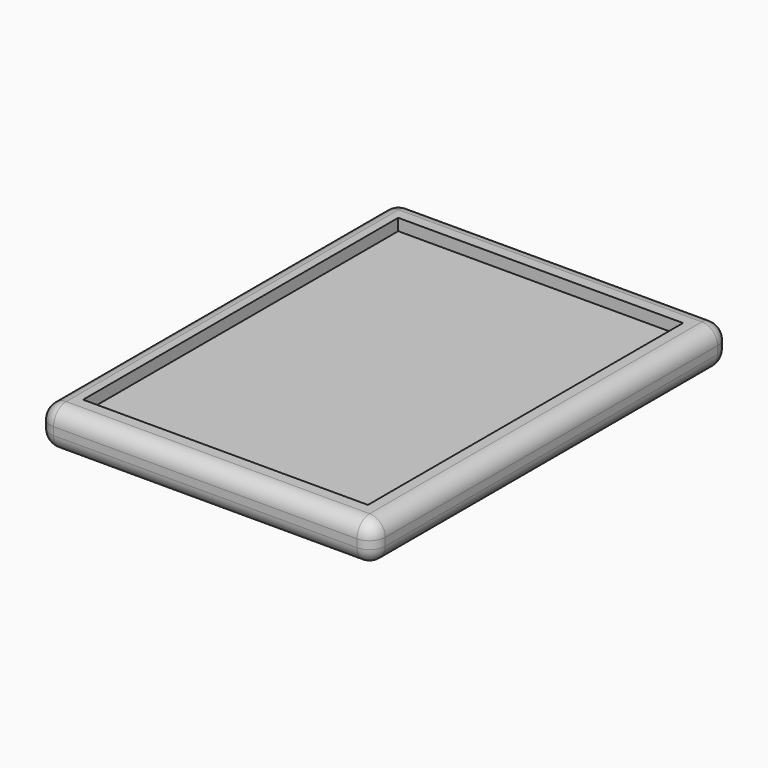
from build123d import *

# Parameters (mm, degrees)
F0_W         = 108.4600649774
F0_H         = 144.723303616
F1_DEPTH     = 12.7
F2_W         = 92.2743044794
F2_H         = 127.6071891189
F3_DEPTH     = 3.81
F4_R         = 5.08
F5_T1_DEPTH  = 20.32
F5_S5_W      = 5.08
F5_S5_H      = 5.08
F5_T6_DEPTH  = 5.08
F5_S11_W     = 5.08
F5_S11_H     = 5.08
F5_T12_DEPTH = 5.08
F5_S17_W     = 5.08
F5_S17_H     = 5.08
F5_T18_DEPTH = 5.08
F5_S23_W     = 5.08
F5_S23_H     = 5.08
F5_T24_DEPTH = 5.08
F7_DEPTH     = 5.08
F8_DEPTH     = 5.08
F9_R         = 5.08


# Not quite as in the source:
# - a fillet or chamfer that OpenCascade refuses, or shapes differently, is made with other operations: its cross-section is extruded or revolved along the edge and cut away or added


with BuildPart() as f1:
    # F0 (on Top) → F1 (new body)
    with BuildSketch(Plane.XY):
        with Locations((1.0477285832, -0.3120861948)):
            Rectangle(F0_W, F0_H)
    extrude(amount=F1_DEPTH)

    # F2 (on face) → F3 (cut, symmetric)
    with BuildSketch(Plane.XY.offset(12.7)):
        with Locations((0.7300172001, -0.29200688)):
            Rectangle(F2_W, F2_H)
    extrude(amount=F3_DEPTH, both=True, mode=Mode.SUBTRACT)

    # F4
    f4_edges = [f1.edges().sort_by_distance(p)[0] for p in [
        (1.047729, 72.049566, 12.7),
        (-53.182304, -0.312086, 12.7),
        (55.277761, -0.312086, 12.7),
        (1.047729, -72.673738, 12.7),
    ]]
    fillet(f4_edges, radius=F4_R)

    # F5: fillet of radius 5.08 on 4 edges, made by hand

    # F5_s2 → F5_t1 (cut)
    with BuildSketch(Plane.XY.offset(-12.7)):
        with BuildLine():
            ThreePointArc((-48.1023039055, 72.0495656133), (-51.6944063539, 70.5616680617), (-53.1823039055, 66.9695656133))
            Line((-53.1823039055, 66.9695656133), (-53.1823039055, 72.0495656133))
            Line((-53.1823039055, 72.0495656133), (-48.1023039055, 72.0495656133))
        make_face()
        with BuildLine():
            ThreePointArc((55.2777610719, -67.5937380028), (53.7898635203, -71.1858404512), (50.1977610719, -72.6737380028))
            Line((50.1977610719, -72.6737380028), (55.2777610719, -72.6737380028))
            Line((55.2777610719, -72.6737380028), (55.2777610719, -67.5937380028))
        make_face()
        with BuildLine():
            ThreePointArc((50.1977610719, 72.0495656133), (53.7898635203, 70.5616680617), (55.2777610719, 66.9695656133))
            Line((55.2777610719, 66.9695656133), (55.2777610719, 72.0495656133))
            Line((55.2777610719, 72.0495656133), (50.1977610719, 72.0495656133))
        make_face()
        with BuildLine():
            ThreePointArc((-53.1823039055, -67.5937380028), (-51.6944063539, -71.1858404512), (-48.1023039055, -72.6737380028))
            Line((-48.1023039055, -72.6737380028), (-53.1823039055, -72.6737380028))
            Line((-53.1823039055, -72.6737380028), (-53.1823039055, -67.5937380028))
        make_face()
    extrude(amount=F5_T1_DEPTH, mode=Mode.SUBTRACT)


with BuildPart() as f5_tool4:
    # F5_s5 → F5_t6 (new body)
    with BuildSketch(Plane.YZ.offset(-48.1023039055)):
        with Locations((-70.1337380028, 10.16)):
            Rectangle(F5_S5_W, F5_S5_H)
    extrude(amount=-F5_T6_DEPTH)

    # F5_s7 → F5_t8 (revolve, cut)
    with BuildSketch(Plane(origin=(-48.1023039055, -67.5937380028, 7.62), x_dir=(0, 0.7071067812, -0.7071067812), z_dir=(0, 0.7071067812, 0.7071067812))):
        with BuildLine():
            ThreePointArc((0, -5.08), (5.08, 0), (0, 5.08))
            Line((0, 5.08), (0, -5.08))
        make_face()
    revolve(axis=Axis((-48.1023039055, -67.5937380028, 7.62), (-1, 0, 0)), mode=Mode.SUBTRACT)


with BuildPart() as f1_1:
    add(f1.part)

    # F5_t3: cut F5_tool4
    add(f5_tool4.part, mode=Mode.SUBTRACT)


with BuildPart() as f5_tool10:
    # F5_s11 → F5_t12 (new body)
    with BuildSketch(Plane.XZ.offset(-66.9695656133)):
        with Locations((52.7377610719, 10.16)):
            Rectangle(F5_S11_W, F5_S11_H)
    extrude(amount=-F5_T12_DEPTH)

    # F5_s13 → F5_t14 (revolve, cut)
    with BuildSketch(Plane(origin=(50.1977610719, 66.9695656133, 7.62), x_dir=(-0.7071067812, 0, -0.7071067812), z_dir=(0.7071067812, 0, -0.7071067812))):
        with BuildLine():
            ThreePointArc((0, -5.08), (5.08, 0), (0, 5.08))
            Line((0, 5.08), (0, -5.08))
        make_face()
    revolve(axis=Axis((50.1977610719, 66.9695656133, 7.62), (0, 1, 0)), mode=Mode.SUBTRACT)


with BuildPart() as f1_2:
    add(f1_1.part)

    # F5_t9: cut F5_tool10
    add(f5_tool10.part, mode=Mode.SUBTRACT)


with BuildPart() as f5_tool16:
    # F5_s17 → F5_t18 (new body)
    with BuildSketch(Plane.YZ.offset(50.1977610719)):
        with Locations((-70.1337380028, 10.16)):
            Rectangle(F5_S17_W, F5_S17_H)
    extrude(amount=F5_T18_DEPTH)

    # F5_s19 → F5_t20 (revolve, cut)
    with BuildSketch(Plane(origin=(50.1977610719, -67.5937380028, 7.62), x_dir=(0, 0.7071067812, -0.7071067812), z_dir=(0, -0.7071067812, -0.7071067812))):
        with BuildLine():
            ThreePointArc((0, -5.08), (5.08, 0), (0, 5.08))
            Line((0, 5.08), (0, -5.08))
        make_face()
    revolve(axis=Axis((50.1977610719, -67.5937380028, 7.62), (1, 0, 0)), mode=Mode.SUBTRACT)


with BuildPart() as f1_3:
    add(f1_2.part)

    # F5_t15: cut F5_tool16
    add(f5_tool16.part, mode=Mode.SUBTRACT)


with BuildPart() as f5_tool22:
    # F5_s23 → F5_t24 (new body)
    with BuildSketch(Plane.XZ.offset(-66.9695656133)):
        with Locations((-50.6423039055, 10.16)):
            Rectangle(F5_S23_W, F5_S23_H)
    extrude(amount=-F5_T24_DEPTH)

    # F5_s25 → F5_t26 (revolve, cut)
    with BuildSketch(Plane(origin=(-48.1023039055, 66.9695656133, 7.62), x_dir=(0.7071067812, 0, -0.7071067812), z_dir=(0.7071067812, 0, 0.7071067812))):
        with BuildLine():
            ThreePointArc((0, -5.08), (5.08, 0), (0, 5.08))
            Line((0, 5.08), (0, -5.08))
        make_face()
    revolve(axis=Axis((-48.1023039055, 66.9695656133, 7.62), (0, 1, 0)), mode=Mode.SUBTRACT)


with BuildPart() as f1_4:
    add(f1_3.part)

    # F5_t21: cut F5_tool22
    add(f5_tool22.part, mode=Mode.SUBTRACT)

    # F6 (on face) → F7 (cut)
    with BuildSketch(Plane(origin=(0, 0, 0), x_dir=(1, 0, 0), z_dir=(0, 0, -1))):
        Polygon((3.4059861085, 7.1879082529), (-20.5314729904, -16.2908951516), (-9.6110993139, 46.108120036), (-34.5313920437, 46.108120036), (-35.3613404431, 41.5870853339), (-29.0712052055, 39.9490292824), (-45.1023137626, -50.8866389588), (-26.7560859861, -50.8866389588), (-22.1040067999, -24.7432643772), (-14.7436749419, -19.9601407069), (-3.4083270657, -50.8866389588), (18.0174460877, -50.8866389588), (18.781872245, -46.3874450041), (13.3216854068, -44.7493889526), (-1.8357932562, -8.0132519048), (14.7413339847, 7.2752712423), (21.0314692224, 8.7604420623), (21.7740546324, 13.2814767644), (-1.7047487721, 13.2814767644), (-2.4473341821, 8.7604420623), align=None)
    extrude(amount=-F7_DEPTH, mode=Mode.SUBTRACT)

    # F6 (on face) → F8 (cut)
    with BuildSketch(Plane(origin=(0, 0, 0), x_dir=(1, 0, 0), z_dir=(0, 0, -1))):
        with BuildLine():
            add(Edge.make_bspline(
                [(35.2279550018, -52.874146968), (30.5103535736, -52.874146968), (27.2014803496, -49.598034865)],
                knots=[0, 0, 0, 1, 1, 1], degree=2))
            add(Edge.make_bspline(
                [(43.2653500278, -49.5543533703), (39.9892379248, -52.874146968), (35.2279550018, -52.874146968)],
                knots=[0, 0, 0, 1, 1, 1], degree=2))
            add(Edge.make_bspline(
                [(46.5414621307, -41.5387990917), (46.5414621307, -46.2345597726), (43.2653500278, -49.5543533703)],
                knots=[0, 0, 0, 1, 1, 1], degree=2))
            add(Edge.make_bspline(
                [(43.2325889067, -33.4795633185), (46.5414621307, -36.7556754214), (46.5414621307, -41.5387990917)],
                knots=[0, 0, 0, 1, 1, 1], degree=2))
            add(Edge.make_bspline(
                [(35.2279550018, -30.2034512155), (39.9237156827, -30.2034512155), (43.2325889067, -33.4795633185)],
                knots=[0, 0, 0, 1, 1, 1], degree=2))
            add(Edge.make_bspline(
                [(27.1687192286, -33.5123244395), (30.4448313315, -30.2034512155), (35.2279550018, -30.2034512155)],
                knots=[0, 0, 0, 1, 1, 1], degree=2))
            add(Edge.make_bspline(
                [(23.8926071256, -41.5387990917), (23.8926071256, -36.8211976635), (27.1687192286, -33.5123244395)],
                knots=[0, 0, 0, 1, 1, 1], degree=2))
            add(Edge.make_bspline(
                [(27.2014803496, -49.598034865), (23.8926071256, -46.321922762), (23.8926071256, -41.5387990917)],
                knots=[0, 0, 0, 1, 1, 1], degree=2))
        make_face()
    extrude(amount=-F8_DEPTH, mode=Mode.SUBTRACT)

    # F9
    f9_edges = [f1_4.edges().sort_by_distance(p)[0] for p in [
        (-51.694406, -71.18584, 0),
    ]]
    fillet(f9_edges, radius=F9_R)


solid = f1_4.part
